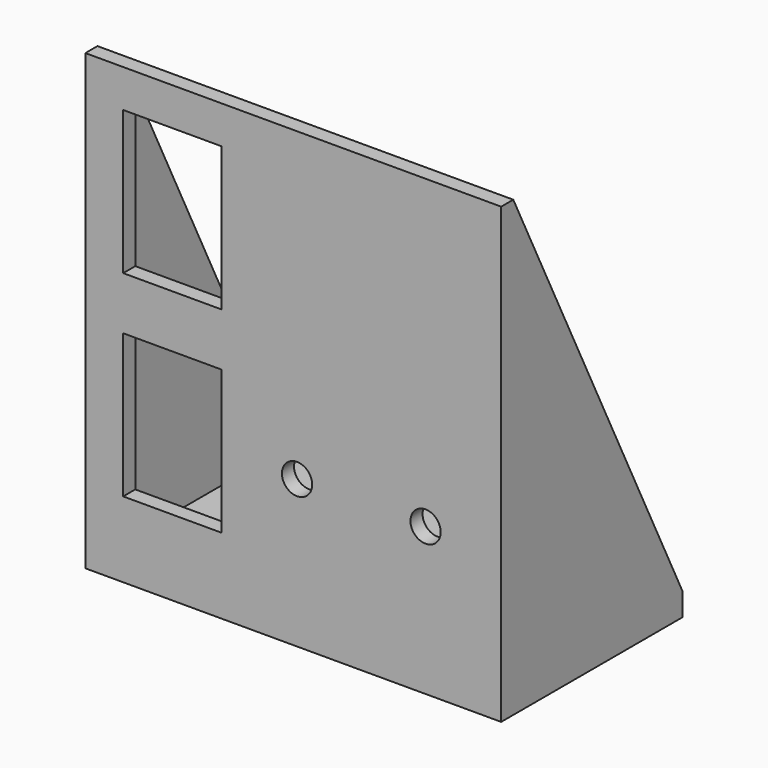
from build123d import *

# Parameters (mm, degrees)
F0_W     = 49
F0_H     = 28
F0_R     = 2.5
F1_DEPTH = 3
F0_W_2   = 3
F0_H_2   = 2
F2_DEPTH = 60
F4_DEPTH = 55
F5_W     = 13
F5_H     = 19
F5_R     = 2
F6_DEPTH = 25


# Not quite as in the source:
# - a feature names something its author has since deleted; it is built from what else it names


with BuildPart() as f1:
    # F0 (on Top) → F1 (new body)
    with BuildSketch(Plane.XY):
        with Locations((0, 1)):
            Rectangle(F0_W, F0_H)
        with Locations((-17.5, 0)):
            Circle(F0_R, mode=Mode.SUBTRACT)
        with Locations((17.5, 0)):
            Circle(F0_R, mode=Mode.SUBTRACT)
    extrude(amount=F1_DEPTH)

    # F0 (on Top) → F2 (join)
    with BuildSketch(Plane.XY):
        with Locations((-26, 1)):
            Rectangle(F0_W_2, F0_H)
        with Locations((-26, -14)):
            Rectangle(F0_W_2, F0_H_2)
        with Locations((0, -14)):
            Rectangle(F0_W, F0_H_2)
        with Locations((26, -14)):
            Rectangle(F0_W_2, F0_H_2)
        with Locations((26, 1)):
            Rectangle(F0_W_2, F0_H)
    extrude(amount=F2_DEPTH)

    # F3 (on face) → F4 (cut)
    with BuildSketch(Plane(origin=(-27.5, 0, 0), x_dir=(0, -1, 0), z_dir=(-1, 0, 0))):
        Polygon((13, 60), (-15, 60), (-15, 3), align=None)
    extrude(amount=-F4_DEPTH, mode=Mode.SUBTRACT)

    # F5 (on face) → F6 (cut)
    with BuildSketch(Plane.XZ.offset(15)):
        Polygon((-22.5, 53), (-22.5, 36), (-9.5, 36), (-9.5, 55), (-22.5, 55), align=None)
        with Locations((-16, 19.5)):
            Rectangle(F5_W, F5_H)
        with Locations((0.5, 19.5)):
            Circle(F5_R)
        with Locations((17.5, 19.5)):
            Circle(F5_R)
    extrude(amount=-F6_DEPTH, mode=Mode.SUBTRACT)


solid = f1.part
